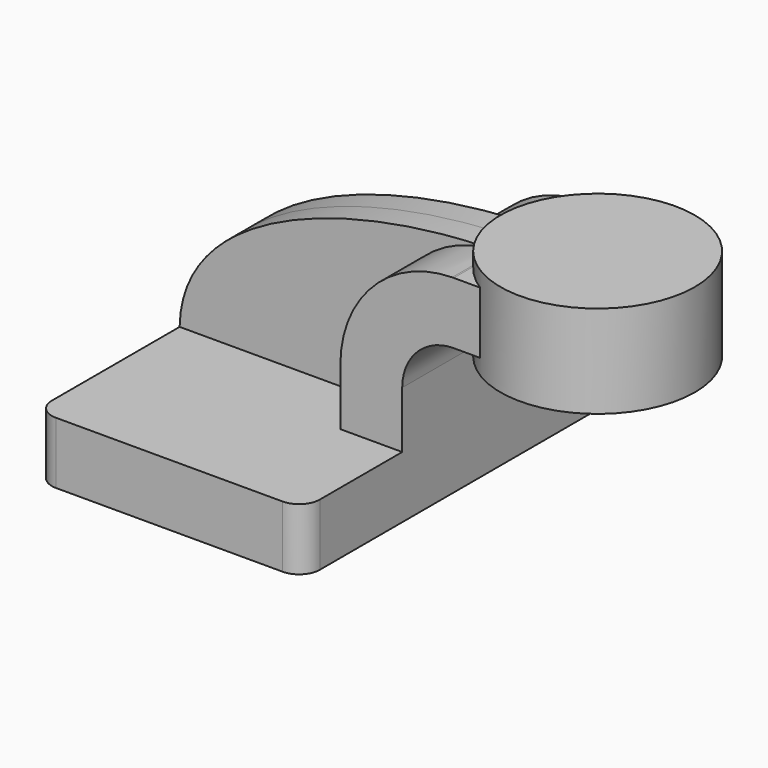
from build123d import *

# Parameters (mm, degrees)
F1_DEPTH = 63.5
F2_DEPTH = 25.4
F3_DEPTH = 7.9375
F4_DEPTH = 25.4
F6_R     = 6.35


# Not quite as in the source:
# - a feature names something its author has since deleted; it is built from what else it names


with BuildPart() as f1:
    # F0 (on Front) → F1 (new body, symmetric)
    with BuildSketch(Plane.XZ):
        Polygon((-41.275, 9.525), (-41.275, -9.525), (41.275, -9.525), (41.275, 9.525), (22.225, 9.525), align=None)
    extrude(amount=F1_DEPTH, both=True)

    # F0 (on Front) → F2 (join, symmetric)
    with BuildSketch(Plane.XZ):
        with BuildLine():
            Line((22.225, 9.525), (41.275, 9.525))
            Line((41.275, 9.525), (41.275, 26.9875))
            ThreePointArc((41.275, 26.9875), (45.9246798487, 38.2128201513), (57.15, 42.8625))
            Line((57.15, 42.8625), (60.325, 42.8625))
            Line((60.325, 42.8625), (60.325, 61.9125))
            Line((60.325, 61.9125), (57.15, 61.9125))
            add(Edge.make_bspline(
                [(56.6876973993, 61.9094401137), (56.8419218796, 61.9106607794), (56.996023665, 61.9116806988), (57.15, 61.9125)],
                knots=[111.1067595469, 111.1067595469, 111.1067595469, 111.1067595469, 111.4985685166, 111.4985685166, 111.4985685166, 111.4985685166], degree=3))
            ThreePointArc((56.6876973993, 61.9094401137), (32.2913843574, 51.5192111783), (22.225, 26.9875))
            Line((22.225, 26.9875), (22.225, 9.525))
        make_face()
    extrude(amount=F2_DEPTH, both=True)

    # F0 (on Front) → F3 (join, symmetric)
    with BuildSketch(Plane.XZ):
        with BuildLine():
            add(Edge.make_bspline(
                [(-41.275, 9.525), (-40.6467419825, 45.0743155721), (12.9536750235, 61.5632913076), (56.6876973993, 61.9094401137)],
                knots=[0, 0, 0, 0, 111.1067595469, 111.1067595469, 111.1067595469, 111.1067595469], degree=3))
            Line((-41.275, 9.525), (22.225, 9.525))
            Line((22.225, 9.525), (22.225, 26.9875))
            ThreePointArc((22.225, 26.9875), (32.2913843574, 51.5192111783), (56.6876973993, 61.9094401137))
        make_face()
    extrude(amount=F3_DEPTH, both=True)

    # F0 (on Front) → F4 (join, symmetric)
    with BuildSketch(Plane.XZ):
        Polygon((81.1691840627, 61.9125), (60.325, 61.9125), (60.325, 42.8625), (81.1691840627, 42.8625), (81.1691840627, 52.7276583016), align=None)
    extrude(amount=F4_DEPTH, both=True)

    # F0 (on Front) → F5 (revolve)
    with BuildSketch(Plane.XZ):
        Polygon((81.1691840627, 66.675), (81.1691840627, 61.9125), (81.1691840627, 52.7276583016), (81.1691840627, 42.8625), (81.1691840627, 38.1), (111.125, 38.1), (111.125, 66.675), align=None)
    revolve(axis=Axis((81.1691840627, 0, 57.3200791508), (0, 0, 1)))

    # F6
    f6_edges = [f1.edges().sort_by_distance(p)[0] for p in [
        (-41.275, -63.5, 0),
        (41.275, -63.5, 0),
        (41.275, 63.5, 0),
        (-41.275, 63.5, 0),
    ]]
    fillet(f6_edges, radius=F6_R)


solid = f1.part
